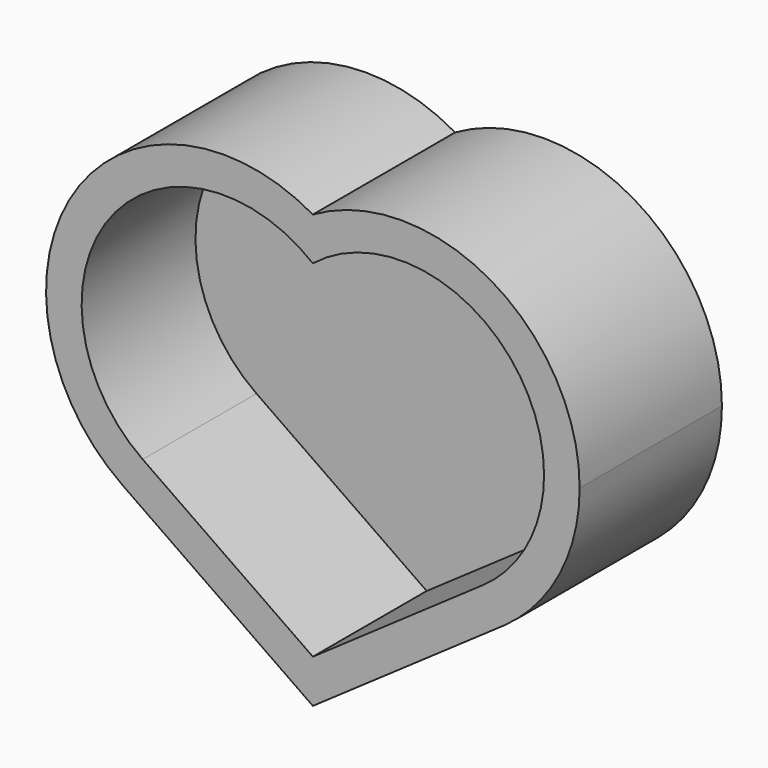
from build123d import *

# Parameters (mm, degrees)
F1_DEPTH = 19.05
F2_DEPTH = 25.4
F3_T     = -5.08


# Not quite as in the source:
# - a feature names something its author has since deleted; it is built from what else it names


with BuildPart() as f1:
    # F0 (on Front) → F1 (new body)
    with BuildSketch(Plane.XZ):
        with BuildLine():
            ThreePointArc((12.7, 21.9970452561), (-21.4428837855, 13.6147983812), (-14.5054559874, -20.8507013455))
            ThreePointArc((-14.5054559874, -20.8507013455), (-1.0693193728, -25.3774812793), (12.7, -21.9970452561))
            ThreePointArc((12.7, -21.9970452561), (0, 0), (12.7, 21.9970452561))
        make_face()
    extrude(amount=F1_DEPTH)

    # F0 (on Front) → F2 (join)
    with BuildSketch(Plane.XZ):
        with BuildLine():
            ThreePointArc((12.7, 21.9970452561), (-21.4428837855, 13.6147983812), (-14.5054559874, -20.8507013455))
            ThreePointArc((-14.5054559874, -20.8507013455), (-1.0693193728, -25.3774812793), (12.7, -21.9970452561))
            ThreePointArc((12.7, -21.9970452561), (0, 0), (12.7, 21.9970452561))
        make_face()
        with BuildLine():
            ThreePointArc((12.7, -21.9970452561), (-1.0693193728, -25.3774812793), (-14.5054559874, -20.8507013455))
            Line((-14.5054559874, -20.8507013455), (12.7, -39.7770452561))
            Line((12.7, -39.7770452561), (12.7, -21.9970452561))
        make_face()
        with BuildLine():
            ThreePointArc((12.7, 21.9970452561), (0, 0), (12.7, -21.9970452561))
            ThreePointArc((12.7, -21.9970452561), (21.9970452561, -12.7), (25.4, 0))
            ThreePointArc((25.4, 0), (21.9970452561, 12.7), (12.7, 21.9970452561))
        make_face()
        with BuildLine():
            ThreePointArc((25.4, 0), (21.9970452561, -12.7), (12.7, -21.9970452561))
            ThreePointArc((12.7, -21.9970452561), (26.4693193728, -25.3774812793), (39.9054559874, -20.8507013455))
            ThreePointArc((39.9054559874, -20.8507013455), (47.9122031583, -11.762682898), (50.8, 0))
            ThreePointArc((50.8, 0), (38.1, 21.9970452561), (12.7, 21.9970452561))
            ThreePointArc((12.7, 21.9970452561), (21.9970452561, 12.7), (25.4, 0))
        make_face()
        with BuildLine():
            ThreePointArc((39.9054559874, -20.8507013455), (26.4693193728, -25.3774812793), (12.7, -21.9970452561))
            Line((12.7, -21.9970452561), (12.7, -39.7770452561))
            Line((12.7, -39.7770452561), (39.9054559874, -20.8507013455))
        make_face()
    extrude(amount=F2_DEPTH)

    # F3
    f3_openings = [f1.faces().sort_by_distance(p)[0] for p in [
        (12.7, -25.4, -2.767667),
    ]]
    offset(amount=F3_T, openings=f3_openings, kind=Kind.INTERSECTION)


solid = f1.part
